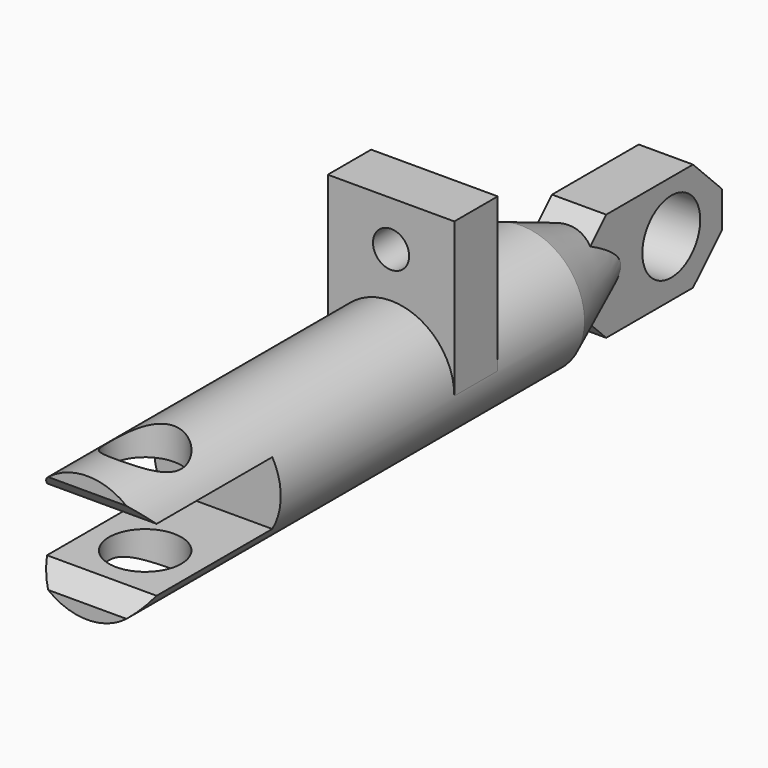
from build123d import *

# Parameters (mm, degrees)
F1_DEPTH     = 1.5
F2_R         = 2
F3_DEPTH     = 3.001
F6_DEPTH     = 30
F7_W         = 14.9228225192
F7_H         = 3.5
F8_DEPTH     = 12.5
F9_W         = 7
F9_H         = 3
F10_DEPTH    = 8.5
F11_R        = 2
F12_DEPTH    = 12.5
F13_R        = 1
F14_DEPTH    = 21.001
F15_T1_DEPTH = 11.2055438024


# Not quite as in the source:
# - a fillet or chamfer that OpenCascade refuses, or shapes differently, is made with other operations: its cross-section is extruded or revolved along the edge and cut away or added


with BuildPart() as f1:
    # F0 (on Right) → F1 (new body, symmetric)
    with BuildSketch(Plane.YZ):
        Polygon((16.8634157784, -1.1044778318), (16.8634157784, 0.8955221682), (14.8634157784, 2.8955221682), (8.8634157784, 2.8955221682), (6.8634157784, 0.8955221682), (6.8634157784, -1.1044778318), (8.8634157784, -3.1044778318), (14.8634157784, -3.1044778318), align=None)
    extrude(amount=F1_DEPTH, both=True)

    # F2 (on face) → F3 (cut, through all)
    with BuildSketch(Plane(origin=(-1.5, 0, 0), x_dir=(0, -1, 0), z_dir=(-1, 0, 0))):
        with Locations((-13.3634157784, 0)):
            Circle(F2_R)
    extrude(amount=-F3_DEPTH, mode=Mode.SUBTRACT)

    # F4 (on Top) → F5 (revolve)
    with BuildSketch(Plane.XY):
        Polygon((0, 4.8634157784), (0, 9.8634157784), (-1.5, 9.8634157784), (-3.5, 4.8634157784), align=None)
    revolve(axis=Axis((0, 7.3634157784, 0), (0, 1, 0)))

    # F6 (add): a face of the model
    f6_faces = [f1.faces().sort_by_distance(p)[0] for p in [
        (0, 4.8634157784, 0),
    ]]
    extrude(f6_faces, amount=F6_DEPTH)

    # F7 (on Right) → F8 (cut, symmetric)
    with BuildSketch(Plane.YZ):
        with Locations((-23.5979954812, 0)):
            Rectangle(F7_W, F7_H)
    extrude(amount=F8_DEPTH, both=True, mode=Mode.SUBTRACT)

    # F9 (on Top) → F10 (join)
    with BuildSketch(Plane.XY):
        with Locations((0, -2.6365842216)):
            Rectangle(F9_W, F9_H)
    extrude(amount=F10_DEPTH)

    # F11 (on Top) → F12 (cut, symmetric)
    with BuildSketch(Plane.XY):
        with Locations((0, -21.1365842216)):
            Circle(F11_R)
    extrude(amount=F12_DEPTH, both=True, mode=Mode.SUBTRACT)

    # F13 (on face) → F14 (cut, through all)
    with BuildSketch(Plane.XZ.offset(4.1365842216)):
        with Locations((0, 6)):
            Circle(F13_R)
    extrude(amount=-F14_DEPTH, mode=Mode.SUBTRACT)

    # F15: chamfer of 1 on 2 edges, made by hand

    # F15_s2 → F15_t1 (cut)
    with BuildSketch(Plane.YZ.offset(-5.6027719012)):
        Polygon((-24.1365842216, -1.75), (-25.1365842216, -2.75), (-25.1365842216, -1.75), align=None)
        Polygon((-24.1365842216, 1.75), (-25.1365842216, 2.75), (-25.1365842216, 1.75), align=None)
    extrude(amount=F15_T1_DEPTH, mode=Mode.SUBTRACT)


solid = f1.part
